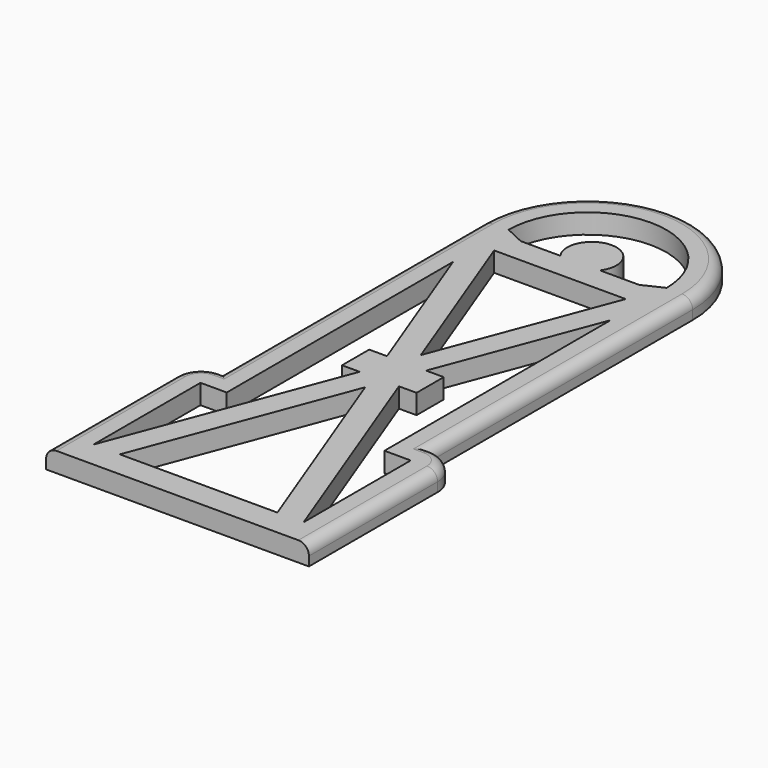
from build123d import *

# Parameters (mm, degrees)
F1_DEPTH     = 3.81
F2_R         = 2.032
F3_T3_ANGLE  = 90
F3_T6_ANGLE  = 90
F3_T9_DEPTH  = 16.51
F3_T12_DEPTH = 16.51


# Not quite as in the source:
# - a fillet or chamfer that OpenCascade refuses, or shapes differently, is made with other operations: its cross-section is extruded or revolved along the edge and cut away or added


with BuildPart() as f1:
    # F0 (on Top) → F1 (new body)
    with BuildSketch(Plane.XY):
        with BuildLine():
            Line((0, 36.1550717625), (0, 0))
            Line((0, 0), (50.8, 0))
            Line((50.8, 0), (50.8, 36.1550717625))
            Line((50.8, 36.1550717625), (45.72, 36.1550717625))
            Line((45.72, 36.1550717625), (45.72, 99.06))
            ThreePointArc((45.72, 99.06), (25.4, 119.38), (5.08, 99.06))
            Line((5.08, 99.06), (5.08, 36.1550717625))
            Line((5.08, 36.1550717625), (0, 36.1550717625))
        make_face()
        Polygon((21.5968196758, 48.7659722567), (5.08, 5.08), (5.08, 30.9497844428), (10.16, 30.9497844428), (10.16, 85.6342857143), (21.623824299, 55.3370357813), (18.1859140491, 55.3370357813), (18.1859140491, 48.7659722567), align=None, mode=Mode.SUBTRACT)
        Polygon((40.64, 5.08), (10.1879829027, 5.08), (25.4079982621, 45.3360045931), align=None, mode=Mode.SUBTRACT)
        Polygon((45.72, 30.9497844428), (45.72, 5.08), (29.1901726596, 48.7659722567), (32.5980894268, 48.7659722567), (32.5980894268, 55.3370357813), (29.1891943801, 55.3370357813), (40.64, 85.6237124205), (40.64, 30.9497844428), align=None, mode=Mode.SUBTRACT)
        Polygon((25.3920017379, 58.8039954069), (12.6709696314, 92.4238659741), (24.3276693245, 92.4238659741), (26.4725103977, 92.4238659741), (38.1030234, 92.4238659741), align=None, mode=Mode.SUBTRACT)
        with BuildLine():
            ThreePointArc((10.16, 99.06), (25.3630832236, 114.3000449305), (40.64, 99.1340130568))
            Line((40.64, 99.1340130568), (36.7868717318, 97.3090561919))
            Line((36.7868717318, 97.3090561919), (29.223334248, 97.3090561919))
            ThreePointArc((29.223334248, 97.3090561919), (25.4000898611, 104.8685646157), (21.5768454742, 97.3090561919))
            Line((21.5768454742, 97.3090561919), (13.8981392212, 97.3090561919))
            Line((13.8981392212, 97.3090561919), (10.16, 99.06))
        make_face(mode=Mode.SUBTRACT)
    extrude(amount=F1_DEPTH)

    # F2
    f2_edges = [f1.edges().sort_by_distance(p)[0] for p in [
        (45.72, 67.607536, 3.81),
        (50.8, 18.077536, 3.81),
        (48.26, 36.155072, 3.81),
        (2.54, 36.155072, 3.81),
        (0, 18.077536, 3.81),
    ]]
    fillet(f2_edges, radius=F2_R)

    # F3: fillet of radius 5.08 on 2 edges, made by hand


with BuildPart() as f3_tool1:
    # F3_s2 → F3_t3 (revolve)
    with BuildSketch(Plane.YZ.offset(5.08)):
        with BuildLine():
            ThreePointArc((34.1230717625, 3.81), (35.5599127419, 3.2148409794), (36.1550717625, 1.778))
            Line((36.1550717625, 1.778), (36.1550717625, 3.81))
            Line((36.1550717625, 3.81), (34.1230717625, 3.81))
        make_face()
    revolve(axis=Axis((5.08, 31.0750717625, 3.81), (0, 0, 1)), revolution_arc=F3_T3_ANGLE)


with BuildPart() as f3_tool4:
    # F3_s5 → F3_t6 (revolve)
    with BuildSketch(Plane.XZ.offset(-31.0750717625)):
        with BuildLine():
            ThreePointArc((48.768, 3.81), (50.2048409794, 3.2148409794), (50.8, 1.778))
            Line((50.8, 1.778), (50.8, 3.81))
            Line((50.8, 3.81), (48.768, 3.81))
        make_face()
    revolve(axis=Axis((45.72, 31.0750717625, 3.81), (0, 0, 1)), revolution_arc=F3_T6_ANGLE)


with BuildPart() as f3_tool7:
    # F3_s8 → F3_t9 (new body)
    with BuildSketch(Plane.XY.offset(-12.7)):
        with BuildLine():
            ThreePointArc((50.8, 31.0750717625), (49.3121024484, 34.667174211), (45.72, 36.1550717625))
            Line((45.72, 36.1550717625), (50.8, 36.1550717625))
            Line((50.8, 36.1550717625), (50.8, 31.0750717625))
        make_face()
    extrude(amount=F3_T9_DEPTH)


with BuildPart() as f3_tool10:
    # F3_s11 → F3_t12 (new body)
    with BuildSketch(Plane.XY.offset(-12.7)):
        with BuildLine():
            ThreePointArc((5.08, 36.1550717625), (1.4878975516, 34.667174211), (0, 31.0750717625))
            Line((0, 31.0750717625), (0, 36.1550717625))
            Line((0, 36.1550717625), (5.08, 36.1550717625))
        make_face()
    extrude(amount=F3_T12_DEPTH)


with BuildPart() as f1_1:
    add(f1.part)

    # F3_t13: cut F3_tool1, F3_tool4, F3_tool7, F3_tool10
    add([f3_tool1.part, f3_tool4.part, f3_tool7.part, f3_tool10.part], mode=Mode.SUBTRACT)


solid = f1_1.part
